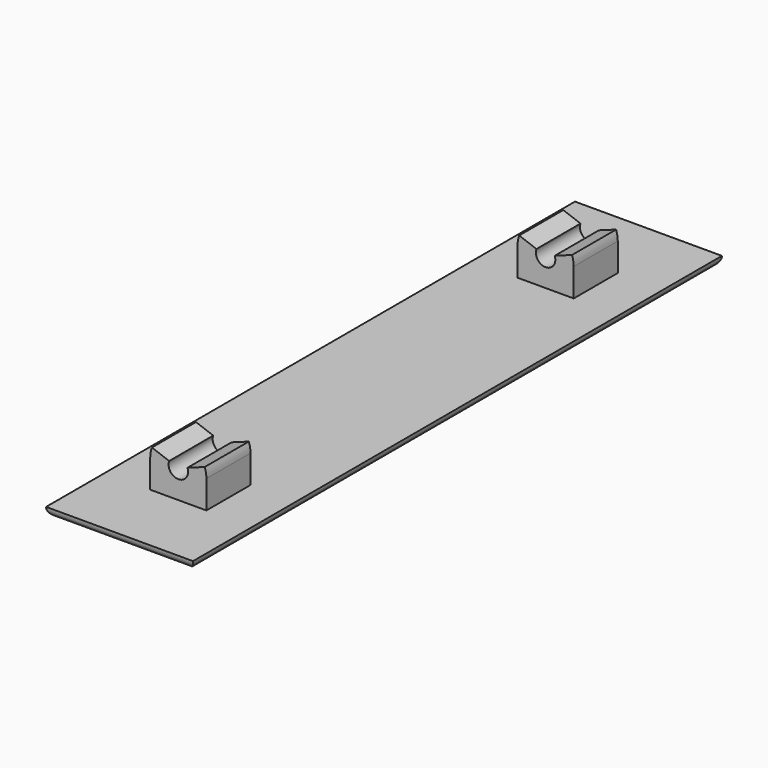
from build123d import *

# Parameters (mm, degrees)
F1_DEPTH = 180
F2_W     = 10.35
F2_H     = 20
F2_H_2   = 110
F3_DEPTH = 25
F4_DEPTH = 25
F5_DEPTH = 25
F6_R     = 2.49999


# Not quite as in the source:
# - a fillet or chamfer is up to 0.001 mm smaller than in the source, because OpenCascade refuses the exact size


with BuildPart() as f1:
    # F0 (on Front) → F1 (new body)
    with BuildSketch(Plane.XZ):
        with BuildLine():
            ThreePointArc((2.4901854451, 0.9063533798), (0, -2.65), (-2.4901854451, 0.9063533798))
            Line((-2.4901854451, 0.9063533798), (-7.188648549, 2.6164540964))
            ThreePointArc((-7.188648549, 2.6164540964), (-7.5337793105, 1.3284085592), (-7.65, 0))
            ThreePointArc((-7.65, 0), (-5.4093668761, -5.4093668761), (0, -7.65))
            ThreePointArc((0, -7.65), (5.4093668761, -5.4093668761), (7.65, 0))
            ThreePointArc((7.65, 0), (7.5337793105, 1.3284085592), (7.188648549, 2.6164540964))
            Line((7.188648549, 2.6164540964), (2.4901854451, 0.9063533798))
        make_face()
        with BuildLine():
            ThreePointArc((0, -7.65), (-5.4093668761, -5.4093668761), (-7.65, 0))
            Line((-7.65, 0), (-7.65, -7.65))
            Line((-7.65, -7.65), (0, -7.65))
        make_face()
        with BuildLine():
            Line((7.65, -7.65), (7.65, 0))
            ThreePointArc((7.65, 0), (5.4093668761, -5.4093668761), (0, -7.65))
            Line((0, -7.65), (7.65, -7.65))
        make_face()
        Polygon((7.65, -7.65), (0, -7.65), (-7.65, -7.65), (-20, -7.65), (-20, -10.15), (20, -10.15), (20, -7.65), align=None)
    extrude(amount=F1_DEPTH)

    # F2 (on face) → F3 (join)
    with BuildSketch(Plane.XY.offset(-7.65)):
        with Locations((14.825, -170)):
            Rectangle(F2_W, F2_H)
        with Locations((14.825, -90)):
            Rectangle(F2_W, F2_H_2)
        with Locations((14.825, -10)):
            Rectangle(F2_W, F2_H)
    extrude(amount=F3_DEPTH)

    # F4 (cut): faces of the model
    f4_faces = [f1.faces().sort_by_distance(p)[0] for p in [
        (9.65, -10, 4.85),
        (9.65, -90, 4.85),
        (9.65, -170, 4.85),
    ]]
    extrude(f4_faces, amount=F4_DEPTH, mode=Mode.SUBTRACT)

    # F5 (cut): faces of the model
    f5_faces = [f1.faces().sort_by_distance(p)[0] for p in [
        (9.65, -10, 4.85),
        (9.65, -90, 4.85),
        (9.65, -170, 4.85),
    ]]
    extrude(f5_faces, amount=-F5_DEPTH, mode=Mode.SUBTRACT)

    # F6 (radius 2.5 in the source; OpenCascade refuses exactly that, so slightly less here)
    f6_edges = [f1.edges().sort_by_distance(p)[0] for p in [
        (-20, -90, -10.15),
        (0, -180, -10.15),
        (20, -90, -10.15),
        (0, 0, -10.15),
    ]]
    fillet(f6_edges, radius=F6_R)


solid = f1.part
